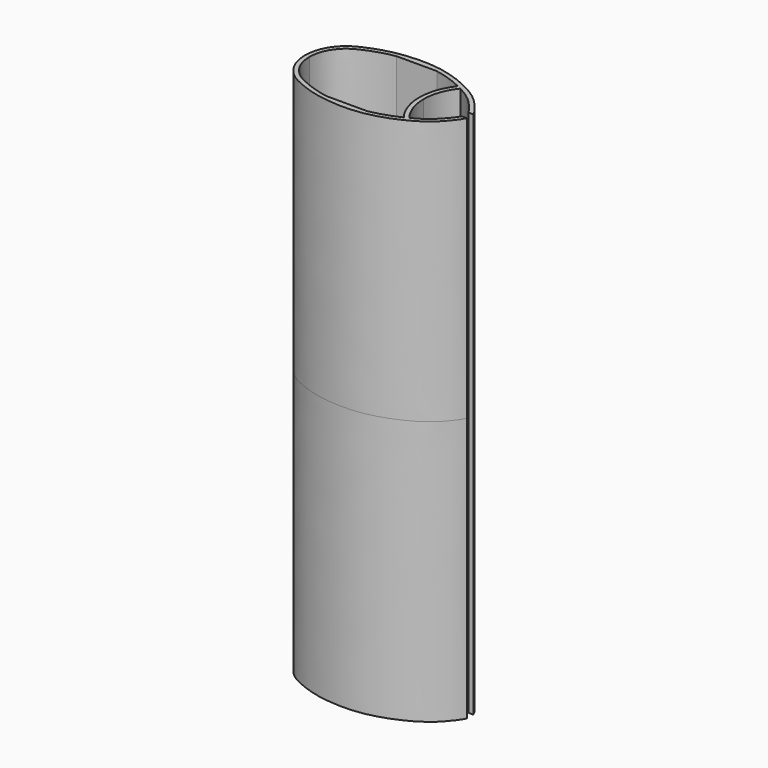
from build123d import *

# Parameters (mm, degrees)
F19_DEPTH = 152.4


# Not quite as in the source:
# - ends of sketch curves that miss each other by under 0.0002 mm in the source are joined
# - the dataset's text gives a spline's control points without its knots; the knots are read off the source's solid


with BuildPart() as f19:
    # F18 (on Top) → F19 (new body, symmetric)
    with BuildSketch(Plane.XY):
        with BuildLine():
            Line((-43.815, 0), (-41.274364031, 0))
            Line((-41.274364031, 0), (-41.274364031, 0.0107594472))
            add(Edge.make_bspline(
                [(-41.274364031, 0.0107594472), (-41.2477378711, 1.3661596464), (-41.0461105432, 3.3581416359), (-40.4801466689, 5.8466573854), (-39.9119087851, 7.6163003428), (-39.2093555266, 9.2678119356), (-38.3748806106, 10.8239592565), (-37.4139591197, 12.2937284374), (-36.3267110013, 13.6931162157), (-35.132922694, 15.0055835598), (-33.8536965602, 16.2044904338), (-32.7323620837, 17.0926256482), (-31.8144631315, 17.7247613585), (-30.8637995003, 18.320756782), (-29.6198390803, 19.0061104284), (-28.309584962, 19.6379349174), (-27.2282396619, 20.1273797903), (-26.1304699992, 20.6115762704), (-24.7648344807, 21.1913224862), (-23.0868238206, 21.8552392863), (-21.3347237158, 22.4913734007), (-19.4620491678, 23.1069136256), (-17.4937213532, 23.686204789), (-15.4662009879, 24.2102580953), (-13.7572955835, 24.586132952), (-12.3927559261, 24.8420192302), (-11.6375273995, 24.9686838433), (-11.2253951687, 25.0334630626), (-11.1550271773, 25.0444)],
                knots=[0.0004181716, 0.0004181716, 0.0004181716, 0.0004181716, 0.03125, 0.046875, 0.0625, 0.078125, 0.09375, 0.109375, 0.125, 0.140625, 0.15625, 0.171875, 0.1796875, 0.1875, 0.203125, 0.21875, 0.2265625, 0.234375, 0.25, 0.265625, 0.28125, 0.296875, 0.3125, 0.328125, 0.34375, 0.3515625, 0.359375, 0.3609843483, 0.3609843483, 0.3609843483, 0.3609843483], degree=3))
            add(Edge.make_bspline(
                [(-11.1550271773, 25.0444), (-10.542199434, 25.1396486856), (-9.2507341781, 25.3205491936), (-7.3235060256, 25.5409372807), (-5.4062672912, 25.7225029254), (-3.6259707874, 25.8679167236), (-1.9439119364, 25.9703614265), (-0.3024423735, 26.0267386411), (1.3666901148, 26.0318853631), (3.0841459509, 25.9889379786), (4.8358815804, 25.9022176908), (6.6182508403, 25.7782185761), (8.3995657193, 25.6136085287), (10.204227939, 25.3891398197), (11.4811176273, 25.1813705052), (12.1601242469, 25.054374244), (12.212939209, 25.0444)],
                knots=[0.3609843483, 0.3609843483, 0.3609843483, 0.3609843483, 0.375, 0.390625, 0.40625, 0.421875, 0.4375, 0.453125, 0.46875, 0.484375, 0.5, 0.515625, 0.53125, 0.546875, 0.5625, 0.5638155672, 0.5638155672, 0.5638155672, 0.5638155672], degree=3))
            add(Edge.make_bspline(
                [(12.212939209, 25.0444), (12.7874079098, 24.935910081), (14.0101485763, 24.6812380165), (15.9013332093, 24.223185306), (17.8100208417, 23.7035416368), (19.6174982681, 23.1637186381), (21.2739675555, 22.6248092168), (22.8673765228, 22.055473021), (24.4716753523, 21.4292847031), (26.1728368077, 20.713506069), (27.630108265, 20.0623448256), (28.4926410945, 19.6608053042), (28.7844012144, 19.5230914963)],
                knots=[0.5638155672, 0.5638155672, 0.5638155672, 0.5638155672, 0.578125, 0.59375, 0.609375, 0.625, 0.640625, 0.65625, 0.671875, 0.6875, 0.703125, 0.7112622913, 0.7112622913, 0.7112622913, 0.7112622913], degree=3))
            add(Edge.make_bspline(
                [(28.7844012144, 19.5230914963), (29.0528707495, 19.3963710863), (29.5952084994, 19.137073037), (30.3776220144, 18.752869828), (30.8778676399, 18.5002539174), (31.1178905157, 18.3771670078)],
                knots=[0.7112622913, 0.7112622913, 0.7112622913, 0.7112622913, 0.71875, 0.7265625, 0.7341002498, 0.7341002498, 0.7341002498, 0.7341002498], degree=3))
            add(Edge.make_bspline(
                [(31.1178905157, 18.3771670078), (31.1266393253, 18.3726805023), (31.632499174, 18.1131209993), (32.5860521639, 17.6068316634), (33.7115864947, 16.9611680115), (34.6154219638, 16.4106109289), (35.5367313786, 15.8276579527), (36.7144333728, 15.0415250136), (37.8645154123, 14.2159344045), (38.733972339, 13.5528506756), (39.5550337441, 12.8979203915), (40.4855128205, 12.0966248777), (41.5131824676, 11.1216924507), (42.5070446229, 10.0950657817), (43.5081058577, 8.991562716), (44.3308167156, 8.0416058596), (44.976892336, 7.278340365), (45.6121545757, 6.5202886328), (46.2066805308, 5.793426823), (46.7687995513, 5.0673381808), (47.1761207946, 4.5162992747), (47.5696893531, 3.9537164713), (47.9591886693, 3.3617532401), (48.2891878893, 2.8316504671), (48.4790184853, 2.5122153516), (48.5516575282, 2.3875989692)],
                knots=[0.7341002498, 0.7341002498, 0.7341002498, 0.7341002498, 0.734375, 0.75, 0.765625, 0.7734375, 0.78125, 0.796875, 0.8125, 0.8203125, 0.828125, 0.84375, 0.859375, 0.875, 0.890625, 0.90625, 0.9140625, 0.921875, 0.9375, 0.9453125, 0.953125, 0.9609375, 0.96875, 0.9765625, 0.9817935421, 0.9817935421, 0.9817935421, 0.9817935421], degree=3))
            Line((48.5516575282, 2.3875989692), (51.435, 2.3875989692))
            add(Edge.make_bspline(
                [(-43.815, 0), (-43.7624752522, 3.0037439428), (-42.7423638876, 8.5233473205), (-39.0064769176, 14.9202682328), (-33.8586937997, 19.8303271293), (-27.9721607189, 22.6424605748), (-21.8677478175, 25.1331163292), (-13.8004564967, 27.3955304745), (-5.8675891054, 28.2786991968), (-0.0489766797, 28.6604633775), (5.9976629011, 28.4342151338), (12.5436865646, 27.7572763922), (19.9604839819, 25.8056227743), (25.5276133686, 23.8341537712), (31.7366717098, 20.9964428844), (36.2360615235, 18.5041540338), (40.964844667, 15.1817120352), (44.1938244908, 12.1020479683), (47.1235637345, 8.7006128803), (49.599038946, 5.6639958266), (51.0575334731, 3.1755801978), (51.435, 2.3875989692)],
                knots=[0, 0, 0, 0, 0.0621231068, 0.1193322831, 0.1753384592, 0.2290296673, 0.2834569581, 0.3451113152, 0.4051603052, 0.456236404, 0.5078123021, 0.5626531156, 0.6210927937, 0.6732906127, 0.7280860429, 0.7768031474, 0.8272977729, 0.8723835911, 0.9169026962, 0.9599145905, 1, 1, 1, 1], degree=3))
        make_face()
        with BuildLine():
            add(Edge.make_bspline(
                [(-11.1550271773, 25.0444), (-10.542199434, 25.1396486856), (-9.2507341781, 25.3205491936), (-7.3235060256, 25.5409372807), (-5.4062672912, 25.7225029254), (-3.6259707874, 25.8679167236), (-1.9439119364, 25.9703614265), (-0.3024423735, 26.0267386411), (1.3666901148, 26.0318853631), (3.0841459509, 25.9889379786), (4.8358815804, 25.9022176908), (6.6182508403, 25.7782185761), (8.3995657193, 25.6136085287), (10.204227939, 25.3891398197), (11.4811176273, 25.1813705052), (12.1601242469, 25.054374244), (12.212939209, 25.0444)],
                knots=[0.3609843483, 0.3609843483, 0.3609843483, 0.3609843483, 0.375, 0.390625, 0.40625, 0.421875, 0.4375, 0.453125, 0.46875, 0.484375, 0.5, 0.515625, 0.53125, 0.546875, 0.5625, 0.5638155672, 0.5638155672, 0.5638155672, 0.5638155672], degree=3))
            Line((-11.1550271773, 25.0444), (12.212939209, 25.0444))
        make_face()
        with BuildLine():
            add(Edge.make_bspline(
                [(28.7844012144, 19.5230914963), (29.0528707495, 19.3963710863), (29.5952084994, 19.137073037), (30.3776220144, 18.752869828), (30.8778676399, 18.5002539174), (31.1178905157, 18.3771670078)],
                knots=[0.7112622913, 0.7112622913, 0.7112622913, 0.7112622913, 0.71875, 0.7265625, 0.7341002498, 0.7341002498, 0.7341002498, 0.7341002498], degree=3))
            ThreePointArc((28.7844012144, 19.5230914963), (23.7973996556, 10.322298401), (22.0726, 0))
            Line((22.0726, 0), (24.6126, 0))
            ThreePointArc((24.6126, 0), (26.2869080345, 9.7472954188), (31.1178905157, 18.3771670078))
        make_face()
    extrude(amount=F19_DEPTH, both=True)

    # F20: F19 across plane


with BuildPart() as f19_1:
    add(f19.part)
    add(f19.part.mirror(Plane.XZ))


solid = f19_1.part
